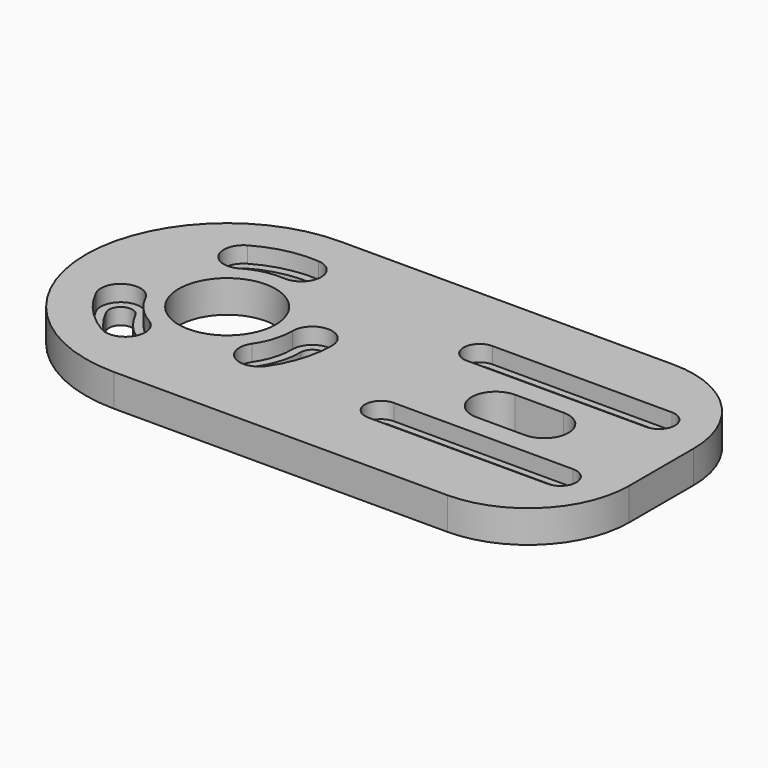
from build123d import *

# Parameters (mm, degrees)
F0_R     = 12
F1_DEPTH = 4
F2_DEPTH = 4


# Not quite as in the source:
# - a feature names something its author has since deleted; it is built from what else it names


with BuildPart() as f1:
    # F0 (on Top) → F1 (new body)
    with BuildSketch(Plane.XY):
        with BuildLine():
            ThreePointArc((64.1499952853, 9.9999063548), (56.8276648149, 27.6775758844), (39.1499952853, 34.9999063548))
            Line((39.1499952853, 34.9999063548), (-43.3500047147, 34.9999063548))
            ThreePointArc((-43.3500047147, 34.9999063548), (-78.3500047147, -9.36452e-05), (-43.3500047147, -35.0000936452))
            Line((-43.3500047147, -35.0000936452), (39.1499952853, -35.0000936452))
            ThreePointArc((39.1499952853, -35.0000936452), (56.8276648149, -27.6777631749), (64.1499952853, -10.0000936452))
            Line((64.1499952853, -10.0000936452), (64.1499952853, 9.9999063548))
        make_face()
        with BuildLine():
            ThreePointArc((-66.7535204548, -11.3259689317), (-64.4773497539, -4.780814469), (-57.9321952912, -7.0569851699))
            ThreePointArc((-57.9321952912, -7.0569851699), (-55.2148750657, -11.0302727714), (-51.4500047147, -14.0297051866))
            ThreePointArc((-51.4500047147, -14.0297051866), (-49.6564802362, -20.7232296651), (-56.3500047147, -22.5167541436))
            ThreePointArc((-56.3500047147, -22.5167541436), (-62.3923892286, -17.7028502675), (-66.7535204548, -11.3259689317))
        make_face(mode=Mode.SUBTRACT)
        with BuildLine():
            ThreePointArc((-21.8397511265, -14.6051951708), (-28.6461065134, -15.9065507518), (-29.9474620944, -9.100195365))
            ThreePointArc((-29.9474620944, -9.100195365), (-27.8651542077, -4.7602832187), (-27.1500047147, -9.36452e-05))
            ThreePointArc((-27.1500047147, -9.36452e-05), (-22.2500047147, 4.8999063548), (-17.3500047147, -9.36452e-05))
            ThreePointArc((-17.3500047147, -9.36452e-05), (-18.4977755059, -7.6399040718), (-21.8397511265, -14.6051951708))
        make_face(mode=Mode.SUBTRACT)
        with BuildLine():
            ThreePointArc((6.9499952853, -19.2000936452), (2.9999952853, -15.2500936452), (6.9499952853, -11.3000936452))
            Line((6.9499952853, -11.3000936452), (29.1499952853, -11.3000936452))
            Line((29.1499952853, -11.3000936452), (51.3499952853, -11.3000936452))
            ThreePointArc((51.3499952853, -11.3000936452), (55.2999952853, -15.2500936452), (51.3499952853, -19.2000936452))
            Line((51.3499952853, -19.2000936452), (29.1499952853, -19.2000936452))
            Line((29.1499952853, -19.2000936452), (6.9499952853, -19.2000936452))
        make_face(mode=Mode.SUBTRACT)
        with Locations((-43.3500047147, -9.36452e-05)):
            Circle(F0_R, mode=Mode.SUBTRACT)
        with BuildLine():
            ThreePointArc((-51.4500047147, 14.0295178961), (-58.1435291933, 15.8230423746), (-56.3500047147, 22.5165668531))
            ThreePointArc((-56.3500047147, 22.5165668531), (-49.1598494096, 25.3424734035), (-41.4567425628, 25.9308831667))
            ThreePointArc((-41.4567425628, 25.9308831667), (-36.9265578769, 20.6870842851), (-42.1703567586, 16.1568995991))
            ThreePointArc((-42.1703567586, 16.1568995991), (-46.9699848708, 15.7902750544), (-51.4500047147, 14.0295178961))
        make_face(mode=Mode.SUBTRACT)
        with BuildLine():
            Line((29.1499952853, 5.9999063548), (35.1499952853, 5.9999063548))
            ThreePointArc((35.1499952853, 5.9999063548), (41.1499952853, -9.36452e-05), (35.1499952853, -6.0000936452))
            Line((35.1499952853, -6.0000936452), (29.1499952853, -6.0000936452))
            Line((29.1499952853, -6.0000936452), (23.1499952853, -6.0000936452))
            ThreePointArc((23.1499952853, -6.0000936452), (17.1499952853, -9.36452e-05), (23.1499952853, 5.9999063548))
            Line((23.1499952853, 5.9999063548), (29.1499952853, 5.9999063548))
        make_face(mode=Mode.SUBTRACT)
        with BuildLine():
            Line((29.1499952853, 11.2999063548), (6.9499952853, 11.2999063548))
            ThreePointArc((6.9499952853, 11.2999063548), (2.9999952853, 15.2499063548), (6.9499952853, 19.1999063548))
            Line((6.9499952853, 19.1999063548), (29.1499952853, 19.1999063548))
            Line((29.1499952853, 19.1999063548), (51.3499952853, 19.1999063548))
            ThreePointArc((51.3499952853, 19.1999063548), (55.2999952853, 15.2499063548), (51.3499952853, 11.2999063548))
            Line((51.3499952853, 11.2999063548), (29.1499952853, 11.2999063548))
        make_face(mode=Mode.SUBTRACT)
        with BuildLine():
            ThreePointArc((-41.4567425628, 25.9308831667), (-49.1598494096, 25.3424734035), (-56.3500047147, 22.5165668531))
            ThreePointArc((-56.3500047147, 22.5165668531), (-58.1435291933, 15.8230423746), (-51.4500047147, 14.0295178961))
            ThreePointArc((-51.4500047147, 14.0295178961), (-46.9699848708, 15.7902750544), (-42.1703567586, 16.1568995991))
            ThreePointArc((-42.1703567586, 16.1568995991), (-36.9265578769, 20.6870842851), (-41.4567425628, 25.9308831667))
        make_face()
        with BuildLine():
            ThreePointArc((-52.4500047147, 15.7615687036), (-56.4114783857, 16.8230423746), (-55.3500047147, 20.7845160456))
            ThreePointArc((-55.3500047147, 20.7845160456), (-48.7129382793, 23.393045169), (-41.602378113, 23.9361926427))
            ThreePointArc((-41.602378113, 23.9361926427), (-38.9212484009, 20.8327198352), (-42.0247212084, 18.1515901231))
            ThreePointArc((-42.0247212084, 18.1515901231), (-47.4168960012, 17.7397032889), (-52.4500047147, 15.7615687036))
        make_face(mode=Mode.SUBTRACT)
        with BuildLine():
            ThreePointArc((-27.1500047147, -9.36452e-05), (-27.8651542077, -4.7602832187), (-29.9474620944, -9.100195365))
            ThreePointArc((-29.9474620944, -9.100195365), (-28.6461065134, -15.9065507518), (-21.8397511265, -14.6051951708))
            ThreePointArc((-21.8397511265, -14.6051951708), (-18.4977755059, -7.6399040718), (-17.3500047147, -9.36452e-05))
            ThreePointArc((-17.3500047147, -9.36452e-05), (-22.2500047147, 4.8999063548), (-27.1500047147, -9.36452e-05))
        make_face()
        with BuildLine():
            ThreePointArc((-23.4943860179, -13.4817258227), (-27.5226371652, -14.2519158604), (-28.292827203, -10.2236647131))
            ThreePointArc((-28.292827203, -10.2236647131), (-25.9534442686, -5.3479609438), (-25.1500047147, -9.36452e-05))
            ThreePointArc((-25.1500047147, -9.36452e-05), (-22.2500047147, 2.8999063548), (-19.3500047147, -9.36452e-05))
            ThreePointArc((-19.3500047147, -9.36452e-05), (-20.4094854451, -7.0522263467), (-23.4943860179, -13.4817258227))
        make_face(mode=Mode.SUBTRACT)
        with BuildLine():
            ThreePointArc((-51.4500047147, -14.0297051866), (-55.2148750657, -11.0302727714), (-57.9321952912, -7.0569851699))
            ThreePointArc((-57.9321952912, -7.0569851699), (-64.4773497539, -4.780814469), (-66.7535204548, -11.3259689317))
            ThreePointArc((-66.7535204548, -11.3259689317), (-62.3923892286, -17.7028502675), (-56.3500047147, -22.5167541436))
            ThreePointArc((-56.3500047147, -22.5167541436), (-49.6564802362, -20.7232296651), (-51.4500047147, -14.0297051866))
        make_face()
        with BuildLine():
            ThreePointArc((-64.9532500133, -10.4547477558), (-63.606128578, -6.5810849105), (-59.7324657328, -7.9282063458))
            ThreePointArc((-59.7324657328, -7.9282063458), (-56.6796738744, -12.3920232808), (-52.4500047147, -15.7617559941))
            ThreePointArc((-52.4500047147, -15.7617559941), (-51.3885310438, -19.7232296651), (-55.3500047147, -20.7847033361))
            ThreePointArc((-55.3500047147, -20.7847033361), (-60.9275904198, -16.3410997581), (-64.9532500133, -10.4547477558))
        make_face(mode=Mode.SUBTRACT)
        with BuildLine():
            ThreePointArc((6.9499952853, 19.1999063548), (2.9999952853, 15.2499063548), (6.9499952853, 11.2999063548))
            Line((6.9499952853, 11.2999063548), (29.1499952853, 11.2999063548))
            Line((29.1499952853, 11.2999063548), (51.3499952853, 11.2999063548))
            ThreePointArc((51.3499952853, 11.2999063548), (55.2999952853, 15.2499063548), (51.3499952853, 19.1999063548))
            Line((51.3499952853, 19.1999063548), (29.1499952853, 19.1999063548))
            Line((29.1499952853, 19.1999063548), (6.9499952853, 19.1999063548))
        make_face()
        with BuildLine():
            Line((29.1499952853, 13.0499063548), (6.9499952853, 13.0499063548))
            ThreePointArc((6.9499952853, 13.0499063548), (4.7499952853, 15.2499063548), (6.9499952853, 17.4499063548))
            Line((6.9499952853, 17.4499063548), (29.1499952853, 17.4499063548))
            Line((29.1499952853, 17.4499063548), (51.3499952853, 17.4499063548))
            ThreePointArc((51.3499952853, 17.4499063548), (53.5499952853, 15.2499063548), (51.3499952853, 13.0499063548))
            Line((51.3499952853, 13.0499063548), (29.1499952853, 13.0499063548))
        make_face(mode=Mode.SUBTRACT)
        with BuildLine():
            Line((29.1499952853, -11.3000936452), (6.9499952853, -11.3000936452))
            ThreePointArc((6.9499952853, -11.3000936452), (2.9999952853, -15.2500936452), (6.9499952853, -19.2000936452))
            Line((6.9499952853, -19.2000936452), (29.1499952853, -19.2000936452))
            Line((29.1499952853, -19.2000936452), (51.3499952853, -19.2000936452))
            ThreePointArc((51.3499952853, -19.2000936452), (55.2999952853, -15.2500936452), (51.3499952853, -11.3000936452))
            Line((51.3499952853, -11.3000936452), (29.1499952853, -11.3000936452))
        make_face()
        with BuildLine():
            ThreePointArc((6.9499952853, -17.4500936452), (4.7499952853, -15.2500936452), (6.9499952853, -13.0500936452))
            Line((6.9499952853, -13.0500936452), (29.1499952853, -13.0500936452))
            Line((29.1499952853, -13.0500936452), (51.3499952853, -13.0500936452))
            ThreePointArc((51.3499952853, -13.0500936452), (53.5499952853, -15.2500936452), (51.3499952853, -17.4500936452))
            Line((51.3499952853, -17.4500936452), (29.1499952853, -17.4500936452))
            Line((29.1499952853, -17.4500936452), (6.9499952853, -17.4500936452))
        make_face(mode=Mode.SUBTRACT)
    extrude(amount=-F1_DEPTH)

    # F0 (on Top) → F2 (join)
    with BuildSketch(Plane.XY):
        with BuildLine():
            ThreePointArc((64.1499952853, 9.9999063548), (56.8276648149, 27.6775758844), (39.1499952853, 34.9999063548))
            Line((39.1499952853, 34.9999063548), (-43.3500047147, 34.9999063548))
            ThreePointArc((-43.3500047147, 34.9999063548), (-78.3500047147, -9.36452e-05), (-43.3500047147, -35.0000936452))
            Line((-43.3500047147, -35.0000936452), (39.1499952853, -35.0000936452))
            ThreePointArc((39.1499952853, -35.0000936452), (56.8276648149, -27.6777631749), (64.1499952853, -10.0000936452))
            Line((64.1499952853, -10.0000936452), (64.1499952853, 9.9999063548))
        make_face()
        with BuildLine():
            ThreePointArc((-66.7535204548, -11.3259689317), (-64.4773497539, -4.780814469), (-57.9321952912, -7.0569851699))
            ThreePointArc((-57.9321952912, -7.0569851699), (-55.2148750657, -11.0302727714), (-51.4500047147, -14.0297051866))
            ThreePointArc((-51.4500047147, -14.0297051866), (-49.6564802362, -20.7232296651), (-56.3500047147, -22.5167541436))
            ThreePointArc((-56.3500047147, -22.5167541436), (-62.3923892286, -17.7028502675), (-66.7535204548, -11.3259689317))
        make_face(mode=Mode.SUBTRACT)
        with BuildLine():
            ThreePointArc((-21.8397511265, -14.6051951708), (-28.6461065134, -15.9065507518), (-29.9474620944, -9.100195365))
            ThreePointArc((-29.9474620944, -9.100195365), (-27.8651542077, -4.7602832187), (-27.1500047147, -9.36452e-05))
            ThreePointArc((-27.1500047147, -9.36452e-05), (-22.2500047147, 4.8999063548), (-17.3500047147, -9.36452e-05))
            ThreePointArc((-17.3500047147, -9.36452e-05), (-18.4977755059, -7.6399040718), (-21.8397511265, -14.6051951708))
        make_face(mode=Mode.SUBTRACT)
        with BuildLine():
            ThreePointArc((6.9499952853, -19.2000936452), (2.9999952853, -15.2500936452), (6.9499952853, -11.3000936452))
            Line((6.9499952853, -11.3000936452), (29.1499952853, -11.3000936452))
            Line((29.1499952853, -11.3000936452), (51.3499952853, -11.3000936452))
            ThreePointArc((51.3499952853, -11.3000936452), (55.2999952853, -15.2500936452), (51.3499952853, -19.2000936452))
            Line((51.3499952853, -19.2000936452), (29.1499952853, -19.2000936452))
            Line((29.1499952853, -19.2000936452), (6.9499952853, -19.2000936452))
        make_face(mode=Mode.SUBTRACT)
        with Locations((-43.3500047147, -9.36452e-05)):
            Circle(F0_R, mode=Mode.SUBTRACT)
        with BuildLine():
            ThreePointArc((-51.4500047147, 14.0295178961), (-58.1435291933, 15.8230423746), (-56.3500047147, 22.5165668531))
            ThreePointArc((-56.3500047147, 22.5165668531), (-49.1598494096, 25.3424734035), (-41.4567425628, 25.9308831667))
            ThreePointArc((-41.4567425628, 25.9308831667), (-36.9265578769, 20.6870842851), (-42.1703567586, 16.1568995991))
            ThreePointArc((-42.1703567586, 16.1568995991), (-46.9699848708, 15.7902750544), (-51.4500047147, 14.0295178961))
        make_face(mode=Mode.SUBTRACT)
        with BuildLine():
            Line((29.1499952853, 5.9999063548), (35.1499952853, 5.9999063548))
            ThreePointArc((35.1499952853, 5.9999063548), (41.1499952853, -9.36452e-05), (35.1499952853, -6.0000936452))
            Line((35.1499952853, -6.0000936452), (29.1499952853, -6.0000936452))
            Line((29.1499952853, -6.0000936452), (23.1499952853, -6.0000936452))
            ThreePointArc((23.1499952853, -6.0000936452), (17.1499952853, -9.36452e-05), (23.1499952853, 5.9999063548))
            Line((23.1499952853, 5.9999063548), (29.1499952853, 5.9999063548))
        make_face(mode=Mode.SUBTRACT)
        with BuildLine():
            Line((29.1499952853, 11.2999063548), (6.9499952853, 11.2999063548))
            ThreePointArc((6.9499952853, 11.2999063548), (2.9999952853, 15.2499063548), (6.9499952853, 19.1999063548))
            Line((6.9499952853, 19.1999063548), (29.1499952853, 19.1999063548))
            Line((29.1499952853, 19.1999063548), (51.3499952853, 19.1999063548))
            ThreePointArc((51.3499952853, 19.1999063548), (55.2999952853, 15.2499063548), (51.3499952853, 11.2999063548))
            Line((51.3499952853, 11.2999063548), (29.1499952853, 11.2999063548))
        make_face(mode=Mode.SUBTRACT)
    extrude(amount=F2_DEPTH)


solid = f1.part
